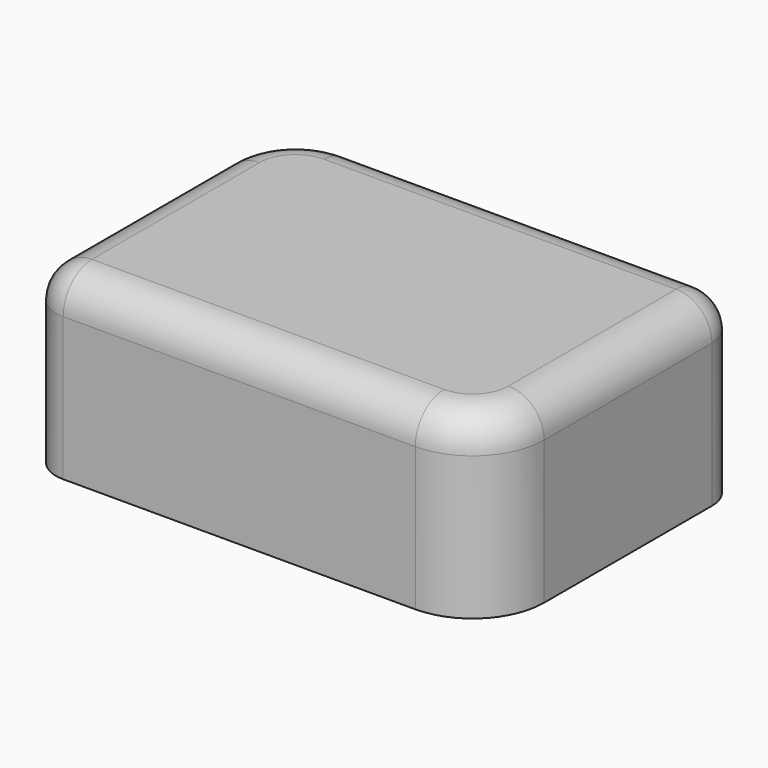
from build123d import *

# Parameters (mm, degrees)
F1_DEPTH    = 25
F2_R        = 5
F3_T1_DEPTH = 32.5
F3_S5_W     = 5
F3_S5_H     = 5
F3_T6_DEPTH = 5


# Not quite as in the source:
# - a fillet or chamfer that OpenCascade refuses, or shapes differently, is made with other operations: its cross-section is extruded or revolved along the edge and cut away or added


with BuildPart() as f1:
    # F0 (on Top) → F1 (new body)
    with BuildSketch(Plane.XY):
        with BuildLine():
            Line((22.5896425545, 23.4159377009), (-31.5712185204, 23.4159377009))
            ThreePointArc((-31.5712185204, 23.4159377009), (-38.6422863323, 20.4870055127), (-41.5712185204, 13.4159377009))
            Line((-41.5712185204, 13.4159377009), (-41.5712185204, -20.8640433848))
            Line((-41.5712185204, -20.8640433848), (12.5896425545, -20.8640433848))
            ThreePointArc((12.5896425545, -20.8640433848), (19.6607103664, -17.9351111967), (22.5896425545, -10.8640433848))
            Line((22.5896425545, -10.8640433848), (22.5896425545, 23.4159377009))
        make_face()
    extrude(amount=F1_DEPTH)

    # F2
    f2_edges = [f1.edges().sort_by_distance(p)[0] for p in [
        (-41.571219, -20.864043, 12.5),
        (-41.571219, -3.724053, 25),
        (-14.490788, -20.864043, 25),
    ]]
    fillet(f2_edges, radius=F2_R)

    # F3: fillet of radius 5 on 1 edges, made by hand

    # F3_s2 → F3_t1 (cut)
    with BuildSketch(Plane.XY.offset(-12.5)):
        with BuildLine():
            ThreePointArc((22.5896425545, 18.4159377009), (21.1251764605, 21.9514716068), (17.5896425545, 23.4159377009))
            Line((17.5896425545, 23.4159377009), (22.5896425545, 23.4159377009))
            Line((22.5896425545, 23.4159377009), (22.5896425545, 18.4159377009))
        make_face()
    extrude(amount=F3_T1_DEPTH, mode=Mode.SUBTRACT)


with BuildPart() as f3_tool4:
    # F3_s5 → F3_t6 (new body)
    with BuildSketch(Plane.YZ.offset(17.5896425545)):
        with Locations((20.9159377009, 22.5)):
            Rectangle(F3_S5_W, F3_S5_H)
    extrude(amount=F3_T6_DEPTH)

    # F3_s7 → F3_t8 (revolve, cut)
    with BuildSketch(Plane(origin=(17.5896425545, 18.4159377009, 20), x_dir=(0, -0.7071067812, -0.7071067812), z_dir=(0, -0.7071067812, 0.7071067812))):
        with BuildLine():
            ThreePointArc((0, -5), (5, 0), (0, 5))
            Line((0, 5), (0, -5))
        make_face()
    revolve(axis=Axis((17.5896425545, 18.4159377009, 20), (1, 0, 0)), mode=Mode.SUBTRACT)


with BuildPart() as f1_1:
    add(f1.part)

    # F3_t3: cut F3_tool4
    add(f3_tool4.part, mode=Mode.SUBTRACT)


solid = f1_1.part
